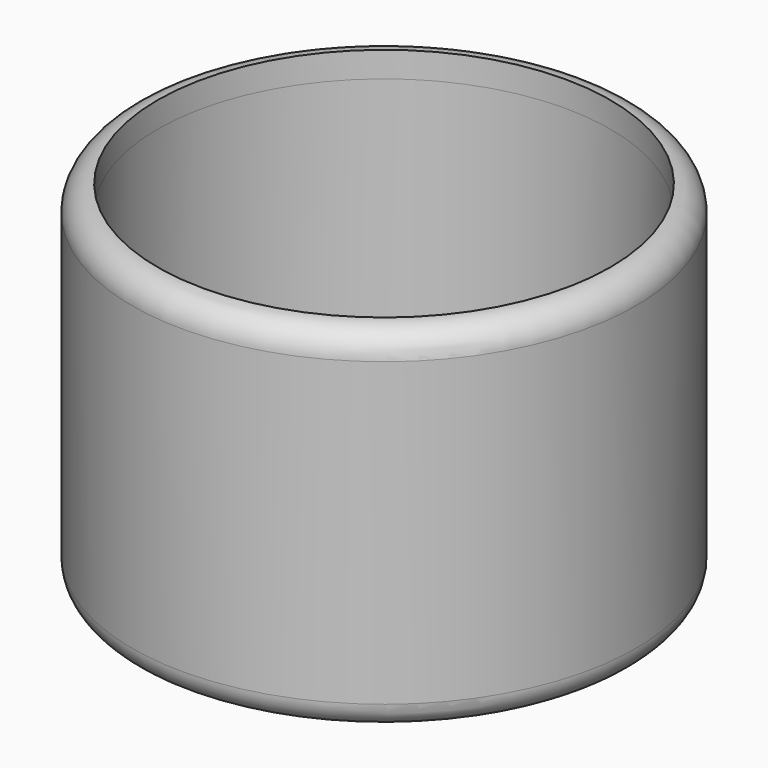
from build123d import *

# Parameters (mm, degrees)
F0_W = 25.0000008
F0_H = 34.99993
F2_R = 2.54
F3_T = -2.54


# Not quite as in the source:
# - a shell that OpenCascade refuses in one call is made with other operations: the cavity is built on its own and cut out


with BuildPart() as f1:
    # F0 (on Front) → F1 (revolve)
    with BuildSketch(Plane.XZ):
        with Locations((-12.5000004, -15.8916468867)):
            Rectangle(F0_W, F0_H)
    revolve(axis=Axis((0, 0, -15.8916468867), (0, 0, -1)))

    # F2
    f2_edges = [f1.edges().sort_by_distance(p)[0] for p in [
        (25.000001, 0, 1.608318),
        (25.000001, 0, -33.391612),
    ]]
    fillet(f2_edges, radius=F2_R)

    # F3: a shell. OpenCascade refuses it in one call, so the cavity is built on its own and cut out:
    # the body offset inwards by the wall thickness, plus a prism from it out through each open face.
    f3_core = offset(f1.part, amount=F3_T, kind=Kind.INTERSECTION, mode=Mode.PRIVATE)
    f3_exits = [f3_core.faces().sort_by_distance(p)[0] for p in [
        (0, 0, -0.931682),
    ]]
    add(f3_core, mode=Mode.SUBTRACT)
    extrude(f3_exits, amount=-F3_T, mode=Mode.SUBTRACT)


solid = f1.part
